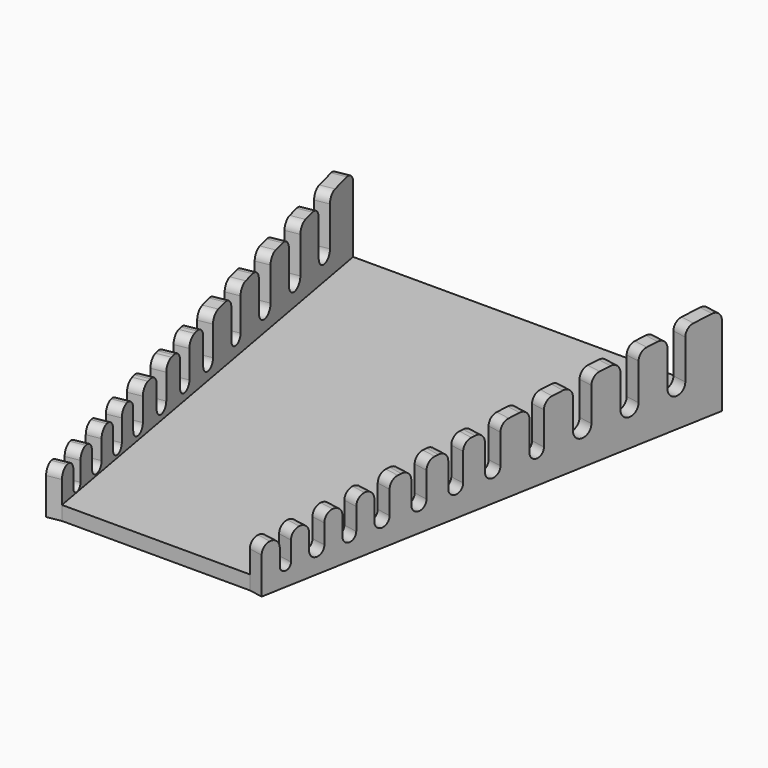
from build123d import *

# Parameters (mm, degrees)
F1_DEPTH = 4.7625
F3_DEPTH = 4.7625


# Not quite as in the source:
# - a length typed as a fraction of an inch, garbled in the dataset ("3 / 203.2 mm" for 3/8 in), is restored


with BuildPart() as f1:
    # F0 (on Top) → F1 (new body)
    with BuildSketch(Plane.XY):
        Polygon((-60.325, 158.75), (-31.75, 0), (31.75, 0), (60.325, 158.75), align=None)
    extrude(amount=F1_DEPTH)


with BuildPart() as f3:
    # F2 (on face) → F3 (new body)
    with BuildSketch(Plane(origin=(30.7535838822, -5.5356450988, 0), x_dir=(0.1771529983, 0.984183324, 0), z_dir=(0.984183324, -0.1771529983, 0))):
        with BuildLine():
            Line((5.6246076965, 12.3508393112), (5.6246076965, 0))
            Line((5.6246076965, 0), (166.9258573042, 0))
            Line((166.9258573042, 0), (166.9258573042, 26.9908811569))
            ThreePointArc((166.9258573042, 26.9908811569), (165.8877258376, 29.3391609254), (163.4522082515, 30.1518040828))
            Line((163.4522082515, 30.1518040828), (156.9639586438, 29.5387838845))
            ThreePointArc((156.9639586438, 29.5387838845), (154.914327928, 28.514729492), (154.0876076965, 26.3778609586))
            Line((154.0876076965, 26.3778609586), (154.0876076965, 13.0153654735))
            ThreePointArc((154.0876076965, 13.0153654735), (150.9761076965, 9.9038654735), (147.8646076965, 13.0153654735))
            Line((147.8646076965, 13.0153654735), (147.8646076965, 25.1899438131))
            ThreePointArc((147.8646076965, 25.1899438131), (146.8264762299, 27.5382235816), (144.3909586438, 28.350866739))
            Line((144.3909586438, 28.350866739), (140.5809586438, 27.9908918464))
            ThreePointArc((140.5809586438, 27.9908918464), (138.531327928, 26.9668374539), (137.7046076965, 24.8299689205))
            Line((137.7046076965, 24.8299689205), (137.7046076965, 12.4694031844))
            ThreePointArc((137.7046076965, 12.4694031844), (134.5296076965, 9.2944031844), (131.3546076965, 12.4694031844))
            Line((131.3546076965, 12.4694031844), (131.3546076965, 23.6300526119))
            ThreePointArc((131.3546076965, 23.6300526119), (130.3164762299, 25.9783323804), (127.8809586438, 26.7909755378))
            Line((127.8809586438, 26.7909755378), (124.0709586438, 26.4310006452))
            ThreePointArc((124.0709586438, 26.4310006452), (122.021327928, 25.4069462527), (121.1946076965, 23.2700777194))
            Line((121.1946076965, 23.2700777194), (121.1946076965, 11.9187342862))
            ThreePointArc((121.1946076965, 11.9187342862), (117.9561076965, 8.6802342862), (114.7176076965, 11.9187342862))
            Line((114.7176076965, 11.9187342862), (114.7176076965, 22.0581622477))
            ThreePointArc((114.7176076965, 22.0581622477), (113.6794762299, 24.4064420162), (111.2439586438, 25.2190851736))
            Line((111.2439586438, 25.2190851736), (107.4339586438, 24.859110281))
            ThreePointArc((107.4339586438, 24.859110281), (105.384327928, 23.8350558885), (104.5576076965, 21.6981873551))
            Line((104.5576076965, 21.6981873551), (104.5576076965, 10.6290753335))
            ThreePointArc((104.5576076965, 10.6290753335), (102.0176076965, 8.0890753335), (99.4776076965, 10.6290753335))
            Line((99.4776076965, 10.6290753335), (99.4776076965, 20.6182626774))
            ThreePointArc((99.4776076965, 20.6182626774), (98.4394762299, 22.9665424459), (96.0039586438, 23.7791856033))
            Line((96.0039586438, 23.7791856033), (92.1939586438, 23.4192107107))
            ThreePointArc((92.1939586438, 23.4192107107), (90.144327928, 22.3951563182), (89.3176076965, 20.2582877848))
            Line((89.3176076965, 20.2582877848), (89.3176076965, 10.2478531007))
            ThreePointArc((89.3176076965, 10.2478531007), (86.5871076965, 7.5173531007), (83.8566076965, 10.2478531007))
            Line((83.8566076965, 10.2478531007), (83.8566076965, 19.1423656178))
            ThreePointArc((83.8566076965, 19.1423656178), (82.8184762299, 21.4906453863), (80.3829586438, 22.3032885437))
            Line((80.3829586438, 22.3032885437), (79.1129586438, 22.1832969128))
            ThreePointArc((79.1129586438, 22.1832969128), (77.063327928, 21.1592425203), (76.2366076965, 19.022373987))
            Line((76.2366076965, 19.022373987), (76.2366076965, 9.6406917873))
            ThreePointArc((76.2366076965, 9.6406917873), (73.6331076965, 7.0371917873), (71.0296076965, 9.6406917873))
            Line((71.0296076965, 9.6406917873), (71.0296076965, 17.9304501461))
            ThreePointArc((71.0296076965, 17.9304501461), (69.9914762299, 20.2787299146), (67.5559586438, 21.091373072))
            Line((67.5559586438, 21.091373072), (66.2859586438, 20.9713814412))
            ThreePointArc((66.2859586438, 20.9713814412), (64.236327928, 19.9473270486), (63.4096076965, 17.8104585153))
            Line((63.4096076965, 17.8104585153), (63.4096076965, 9.2265145536))
            ThreePointArc((63.4096076965, 9.2265145536), (60.7426076965, 6.5595145536), (58.0756076965, 9.2265145536))
            Line((58.0756076965, 9.2265145536), (58.0756076965, 16.7065355114))
            ThreePointArc((58.0756076965, 16.7065355114), (57.0374762299, 19.0548152799), (54.6019586438, 19.8674584373))
            Line((54.6019586438, 19.8674584373), (53.3319586438, 19.7474668064))
            ThreePointArc((53.3319586438, 19.7474668064), (51.282327928, 18.7234124139), (50.4556076965, 16.5865438805))
            Line((50.4556076965, 16.5865438805), (50.4556076965, 8.7464404235))
            ThreePointArc((50.4556076965, 8.7464404235), (47.7886076965, 6.0794404235), (45.1216076965, 8.7464404235))
            Line((45.1216076965, 8.7464404235), (45.1216076965, 15.4826208766))
            ThreePointArc((45.1216076965, 15.4826208766), (44.0834762299, 17.8309006451), (41.6479586438, 18.6435438025))
            ThreePointArc((41.6479586438, 18.6435438025), (39.598327928, 17.61948941), (38.7716076965, 15.4826208766))
            Line((38.7716076965, 15.4826208766), (38.7716076965, 8.0686712363))
            ThreePointArc((38.7716076965, 8.0686712363), (36.3586076965, 5.6556712363), (33.9456076965, 8.0686712363))
            Line((33.9456076965, 8.0686712363), (33.9456076965, 14.4266945251))
            ThreePointArc((33.9456076965, 14.4266945251), (32.9074762299, 16.7749742936), (30.4719586438, 17.5876174509))
            ThreePointArc((30.4719586438, 17.5876174509), (28.422327928, 16.5635630584), (27.5956076965, 14.4266945251))
            Line((27.5956076965, 14.4266945251), (27.5956076965, 7.8992507823))
            ThreePointArc((27.5956076965, 7.8992507823), (24.9286076965, 5.2322507823), (22.2616076965, 7.8992507823))
            Line((22.2616076965, 7.8992507823), (22.2616076965, 13.3227715212))
            ThreePointArc((22.2616076965, 13.3227715212), (21.2234762299, 15.6710512897), (18.7879586438, 16.483694447))
            ThreePointArc((18.7879586438, 16.483694447), (16.738327928, 15.4596400545), (15.9116076965, 13.3227715212))
            Line((15.9116076965, 13.3227715212), (15.9116076965, 6.7931495853))
            ThreePointArc((15.9116076965, 6.7931495853), (13.9431076965, 4.8246495853), (11.9746076965, 6.7931495853))
            Line((11.9746076965, 6.7931495853), (11.9746076965, 12.3508393112))
            ThreePointArc((11.9746076965, 12.3508393112), (10.9364762299, 14.6991190797), (8.5009586438, 15.5117622371))
            ThreePointArc((8.5009586438, 15.5117622371), (6.451327928, 14.4877078446), (5.6246076965, 12.3508393112))
        make_face()
    extrude(amount=F3_DEPTH)


with BuildPart() as f4_1:
    # F4: instance of F3
    add(f3.part.mirror(Plane.YZ))


solid = Compound([f1.part, f3.part, f4_1.part])
